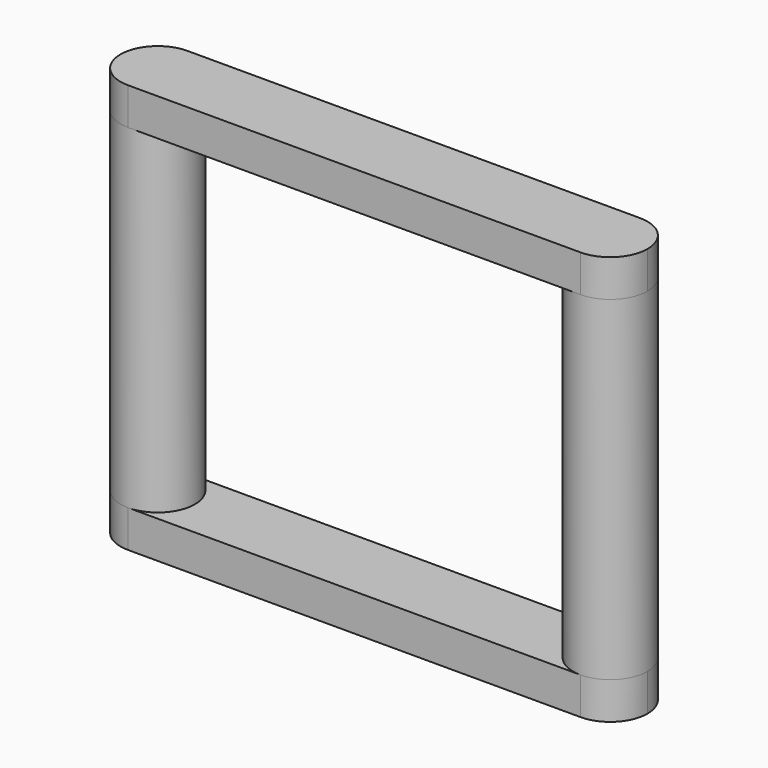
from build123d import *

# Parameters (mm, degrees)
F0_W     = 141.6642213652
F0_H     = 10
F1_DEPTH = 20
F2_R     = 10
F3_DEPTH = 90
F4_W     = 141.6642213652
F4_H     = 20
F5_DEPTH = 10
F6_R     = 9.9999


# Not quite as in the source:
# - a fillet or chamfer is up to 0.001 mm smaller than in the source, because OpenCascade refuses the exact size


with BuildPart() as f1:
    # F0 (on Front) → F1 (new body)
    with BuildSketch(Plane.XZ):
        with Locations((-0.8321106826, -5)):
            Rectangle(F0_W, F0_H)
    extrude(amount=F1_DEPTH)

    # F2 (on face) → F3 (join)
    with BuildSketch(Plane.XY):
        with Locations((-61.6642213652, -10)):
            Circle(F2_R)
        with Locations((60, -10)):
            Circle(F2_R)
    extrude(amount=F3_DEPTH)

    # F4 (on face) → F5 (join)
    with BuildSketch(Plane.XY.offset(90)):
        with Locations((-0.8321106826, -10)):
            Rectangle(F4_W, F4_H)
    extrude(amount=F5_DEPTH)

    # F6 (radius 10 in the source; OpenCascade refuses exactly that, so slightly less here)
    f6_edges = [f1.edges().sort_by_distance(p)[0] for p in [
        (-71.664221, -20, -5),
        (-71.664221, 0, -5),
        (-71.664221, -20, 95),
        (-71.664221, 0, 95),
        (70, 0, 95),
        (70, -20, 95),
        (70, 0, -5),
        (70, -20, -5),
    ]]
    fillet(f6_edges, radius=F6_R)


solid = f1.part
